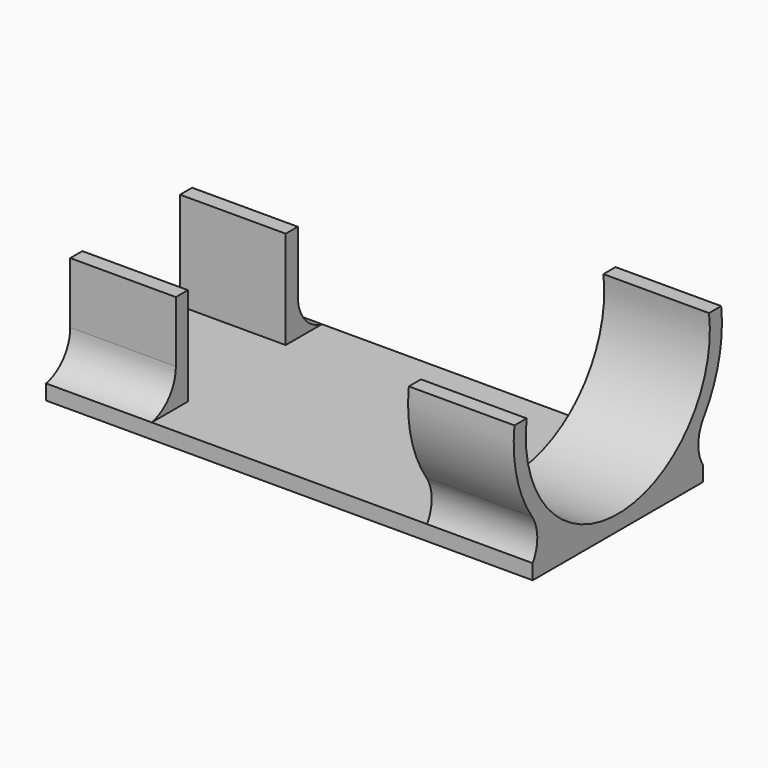
from build123d import *

# Parameters (mm, degrees)
F0_W        = 2
F0_H        = 13
F0_W_2      = 4
F0_H_2      = 2
F1_DEPTH    = 14
F2_DEPTH    = 64.5
F4_DEPTH    = 14
F5_T1_DEPTH = 14
F5_T3_DEPTH = 14


# Not quite as in the source:
# - a fillet or chamfer that OpenCascade refuses, or shapes differently, is made with other operations: its cross-section is extruded or revolved along the edge and cut away or added


with BuildPart() as f1:
    # F0 (on Right) → F1 (new body)
    with BuildSketch(Plane.YZ):
        Polygon((-10.1, 0), (0, 0), (10.1, 0), (10.1, 2), (8.1, 2), (0, 2), (-8.1, 2), (-10.1, 2), align=None)
        with Locations((-9.1, 8.5)):
            Rectangle(F0_W, F0_H)
        with Locations((9.1, 8.5)):
            Rectangle(F0_W, F0_H)
        with Locations((-12.1, 1)):
            Rectangle(F0_W_2, F0_H_2)
        with Locations((12.1, 1)):
            Rectangle(F0_W_2, F0_H_2)
    extrude(amount=F1_DEPTH)

    # F0 (on Right) → F2 (join)
    with BuildSketch(Plane.YZ):
        with Locations((-12.1, 1)):
            Rectangle(F0_W_2, F0_H_2)
        Polygon((-10.1, 0), (0, 0), (10.1, 0), (10.1, 2), (8.1, 2), (0, 2), (-8.1, 2), (-10.1, 2), align=None)
        with Locations((12.1, 1)):
            Rectangle(F0_W_2, F0_H_2)
    extrude(amount=F2_DEPTH)

    # F3 (on face) → F4 (join)
    with BuildSketch(Plane.YZ.offset(64.5)):
        with BuildLine():
            ThreePointArc((15.1106605022, 19.3068031473), (0, 2), (-15.1106605022, 19.3068031473))
            Line((-15.1106605022, 19.3068031473), (-17.1269396219, 19.3068031473))
            ThreePointArc((-17.1269396219, 19.3068031473), (0, 0), (17.1269396219, 19.3068031473))
            Line((17.1269396219, 19.3068031473), (15.1106605022, 19.3068031473))
        make_face()
    extrude(amount=-F4_DEPTH)

    # F5: fillet of radius 5 on 4 edges, made by hand

    # F5_s2 → F5_t1 (join)
    with BuildSketch(Plane.YZ):
        with BuildLine():
            ThreePointArc((-10.1, 6.8989794856), (-11.2270166538, 3.7367018254), (-14.1, 2))
            Line((-14.1, 2), (-10.1, 2))
            Line((-10.1, 2), (-10.1, 6.8989794856))
        make_face()
        with BuildLine():
            ThreePointArc((10.1, 6.8989794856), (11.2270166538, 3.7367018254), (14.1, 2))
            Line((14.1, 2), (10.1, 2))
            Line((10.1, 2), (10.1, 6.8989794856))
        make_face()
    extrude(amount=F5_T1_DEPTH)

    # F5_s4 → F5_t3 (join)
    with BuildSketch(Plane.YZ.offset(50.5)):
        with BuildLine():
            ThreePointArc((-14.2181121589, 7.4823090427), (-13.3404640704, 4.7587904606), (-14.1, 2))
            Line((-14.1, 2), (-8.0622577483, 2))
            ThreePointArc((-8.0622577483, 2), (-11.4724735306, 4.3680416438), (-14.2181121589, 7.4823090427))
        make_face()
        with BuildLine():
            ThreePointArc((14.2181121589, 7.4823090427), (13.3404640704, 4.7587904606), (14.1, 2))
            Line((14.1, 2), (8.0622577483, 2))
            ThreePointArc((8.0622577483, 2), (11.4724735306, 4.3680416438), (14.2181121589, 7.4823090427))
        make_face()
    extrude(amount=F5_T3_DEPTH)


solid = f1.part
